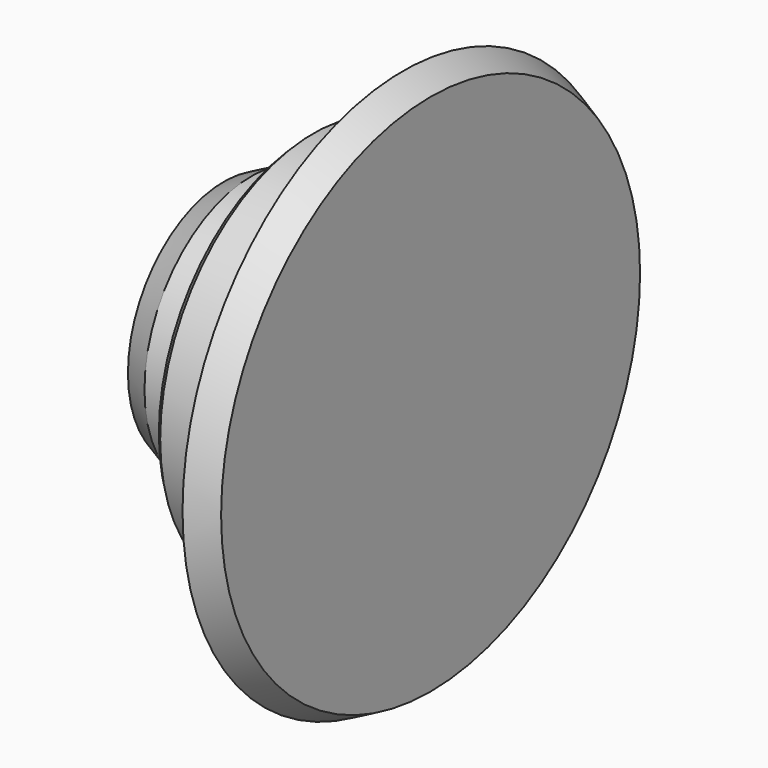
from build123d import *

# Parameters (mm, degrees)
F0_R       = 10
F1_DEPTH   = 4
F2_R       = 4.85
F3_DEPTH   = 3.5
F4_R       = 6.95
F4_R_2     = 6
F5_DEPTH   = 0.5
F6_R       = 10
F6_R_2     = 6.95
F7_DEPTH   = 3
F8_SIZE    = 0.25
F9_SIZE2   = 0.99999
F9_SIZE    = 0.49999
F9_2_SIZE2 = 1
F9_2_SIZE  = 0.5


# Not quite as in the source:
# - a fillet or chamfer is up to 0.001 mm smaller than in the source, because OpenCascade refuses the exact size


with BuildPart() as f1:
    # F0 (on Right) → F1 (new body)
    with BuildSketch(Plane.YZ):
        Circle(F0_R)
    extrude(amount=F1_DEPTH)

    # F2 (on face) → F3 (join)
    with BuildSketch(Plane(origin=(0, 0, 0), x_dir=(0, -1, 0), z_dir=(-1, 0, 0))):
        Circle(F2_R)
    extrude(amount=F3_DEPTH)

    # F4 (on face) → F5 (join)
    with BuildSketch(Plane(origin=(0, 0, 0), x_dir=(0, -1, 0), z_dir=(-1, 0, 0))):
        Circle(F4_R)
        Circle(F4_R_2, mode=Mode.SUBTRACT)
    extrude(amount=F5_DEPTH)

    # F6 (on face) → F7 (cut)
    with BuildSketch(Plane(origin=(0, 0, 0), x_dir=(0, -1, 0), z_dir=(-1, 0, 0))):
        Circle(F6_R)
        Circle(F6_R_2, mode=Mode.SUBTRACT)
    extrude(amount=-F7_DEPTH, mode=Mode.SUBTRACT)

    # F8
    f8_edges = [f1.edges().sort_by_distance(p)[0] for p in [
        (-0.5, 6.95, 0),
        (-0.5, 6, 0),
    ]]
    chamfer(f8_edges, length=F8_SIZE)

    # F9 (size 0.5 and 1 in the source; OpenCascade refuses exactly that, so slightly less here)
    f9_edges = [f1.edges().sort_by_distance(p)[0] for p in [
        (4, -10, 0),
    ]]
    f9_side = f1.faces().sort_by_distance((4, 0, 0))[0]
    chamfer(f9_edges, length=F9_SIZE, length2=F9_SIZE2, reference=f9_side)

    # F9#2
    f9_2_edges = [f1.edges().sort_by_distance(p)[0] for p in [
        (-3.5, 4.85, 0),
    ]]
    f9_2_side = f1.faces().sort_by_distance((-3.5, 0, 0))[0]
    chamfer(f9_2_edges, length=F9_2_SIZE, length2=F9_2_SIZE2, reference=f9_2_side)


solid = f1.part
